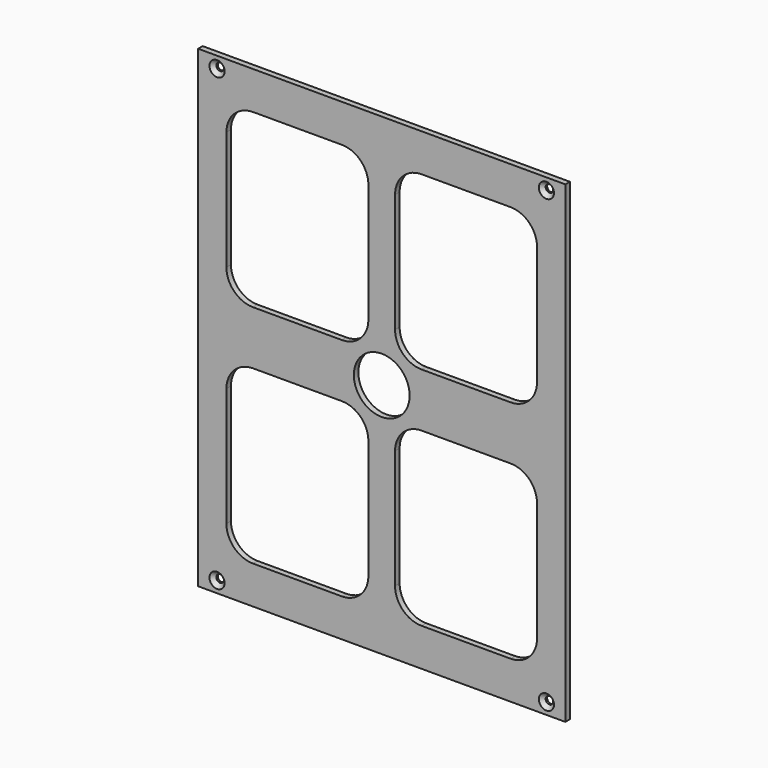
from build123d import *

# Parameters (mm, degrees)
F0_W           = 97
F0_H           = 125
F0_R           = 7.367785
F1_DEPTH       = 1.5
F3_D           = 2
F3_CSINK_D     = 4
F3_CSINK_ANGLE = 90


# Not quite as in the source:
# - a feature names something its author has since deleted; it is built from what else it names


with BuildPart() as f1:
    # F0 (on Front) → F1 (new body)
    with BuildSketch(Plane.XZ):
        Rectangle(F0_W, F0_H)
        with BuildLine():
            Line((-34.0249225795, -7.10684), (-10.5249225795, -7.10684))
            ThreePointArc((-10.5249225795, -7.10684), (-5.5751751112, -9.1570925317), (-3.5249225795, -14.10684))
            Line((-3.5249225795, -14.10684), (-3.5249225795, -45.5))
            ThreePointArc((-3.5249225795, -45.5), (-5.5751751112, -50.4497474683), (-10.5249225795, -52.5))
            Line((-10.5249225795, -52.5), (-34.0249225795, -52.5))
            ThreePointArc((-34.0249225795, -52.5), (-38.9746700478, -50.4497474683), (-41.0249225795, -45.5))
            Line((-41.0249225795, -45.5), (-41.0249225795, -14.10684))
            ThreePointArc((-41.0249225795, -14.10684), (-38.9746700478, -9.1570925317), (-34.0249225795, -7.10684))
        make_face(mode=Mode.SUBTRACT)
        with BuildLine():
            ThreePointArc((41.0249225795, -45.5), (38.9746700478, -50.4497474683), (34.0249225795, -52.5))
            Line((34.0249225795, -52.5), (10.5249225795, -52.5))
            ThreePointArc((10.5249225795, -52.5), (5.5751751112, -50.4497474683), (3.5249225795, -45.5))
            Line((3.5249225795, -45.5), (3.5249225795, -14.10684))
            ThreePointArc((3.5249225795, -14.10684), (5.5751751112, -9.1570925317), (10.5249225795, -7.10684))
            Line((10.5249225795, -7.10684), (34.0249225795, -7.10684))
            ThreePointArc((34.0249225795, -7.10684), (38.9746700478, -9.1570925317), (41.0249225795, -14.10684))
            Line((41.0249225795, -14.10684), (41.0249225795, -45.5))
        make_face(mode=Mode.SUBTRACT)
        with BuildLine():
            ThreePointArc((-3.5249225795, 14.10684), (-5.5751751112, 9.1570925317), (-10.5249225795, 7.10684))
            Line((-10.5249225795, 7.10684), (-34.0249225795, 7.10684))
            ThreePointArc((-34.0249225795, 7.10684), (-38.9746700478, 9.1570925317), (-41.0249225795, 14.10684))
            Line((-41.0249225795, 14.10684), (-41.0249225795, 45.5))
            ThreePointArc((-41.0249225795, 45.5), (-38.9746700478, 50.4497474683), (-34.0249225795, 52.5))
            Line((-34.0249225795, 52.5), (-10.5249225795, 52.5))
            ThreePointArc((-10.5249225795, 52.5), (-5.5751751112, 50.4497474683), (-3.5249225795, 45.5))
            Line((-3.5249225795, 45.5), (-3.5249225795, 14.10684))
        make_face(mode=Mode.SUBTRACT)
        Circle(F0_R, mode=Mode.SUBTRACT)
        with BuildLine():
            ThreePointArc((10.5249225795, 7.10684), (5.5751751112, 9.1570925317), (3.5249225795, 14.10684))
            Line((3.5249225795, 14.10684), (3.5249225795, 45.5))
            ThreePointArc((3.5249225795, 45.5), (5.5751751112, 50.4497474683), (10.5249225795, 52.5))
            Line((10.5249225795, 52.5), (34.0249225795, 52.5))
            ThreePointArc((34.0249225795, 52.5), (38.9746700478, 50.4497474683), (41.0249225795, 45.5))
            Line((41.0249225795, 45.5), (41.0249225795, 14.10684))
            ThreePointArc((41.0249225795, 14.10684), (38.9746700478, 9.1570925317), (34.0249225795, 7.10684))
            Line((34.0249225795, 7.10684), (10.5249225795, 7.10684))
        make_face(mode=Mode.SUBTRACT)
    extrude(amount=F1_DEPTH)

    # F3 (through all)
    with Locations(Plane.XZ.offset(1.5)):
        with Locations((-43.5, -59.5), (43.5, -59.5), (43.5, 59.5), (-43.5, 59.5)):
            CounterSinkHole(F3_D / 2, F3_CSINK_D / 2, counter_sink_angle=F3_CSINK_ANGLE)


solid = f1.part
